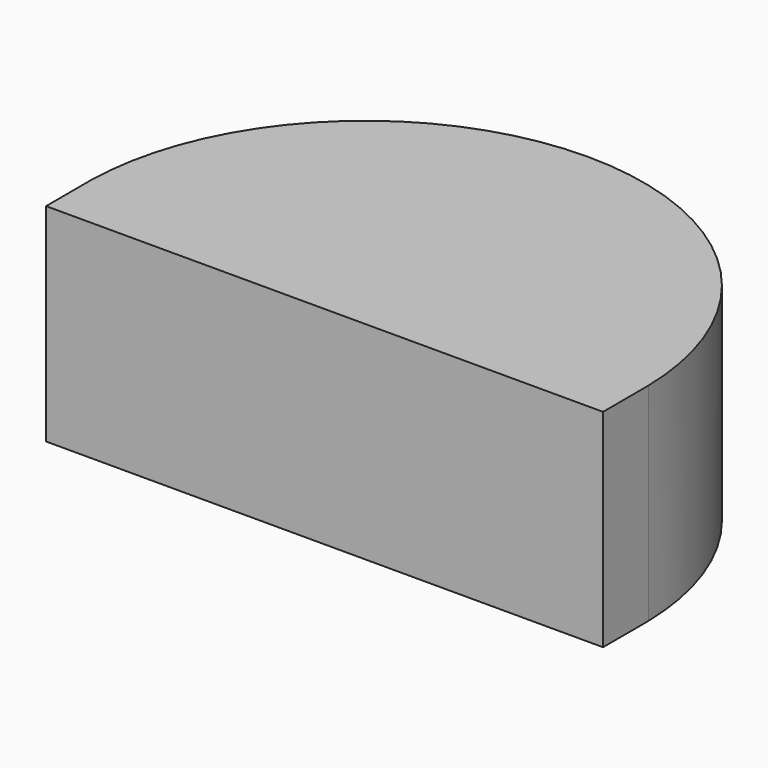
from build123d import *

# Parameters (mm, degrees)
F1_DEPTH = 25.4
F2_W     = 233.7879315019
F2_H     = 188.8666450977
F3_DEPTH = 91.948


# Not quite as in the source:
# - a feature names something its author has since deleted; it is built from what else it names


with BuildPart() as f1:
    # F0 (on Top) → F1 (new body)
    with BuildSketch(Plane.XY):
        with BuildLine():
            ThreePointArc((34.1941267741, -40.3357285894), (0.0107640733, -6.90975175), (-34.0682903974, -40.4420683952))
            Line((-34.0682903974, -40.4420683952), (-33.8233722324, -197.6617082131))
            Line((-33.8233722324, -197.6617082131), (34.4390449391, -197.5553684074))
            Line((34.4390449391, -197.5553684074), (34.1941267741, -40.3357285894))
        make_face()
    extrude(amount=F1_DEPTH)

    # F2 (on face) → F3 (cut)
    with BuildSketch(Plane(origin=(0, 0, 0), x_dir=(1, 0, 0), z_dir=(0, 0, -1))):
        with Locations((-8.5754804313, 141.7237520218)):
            Rectangle(F2_W, F2_H)
    extrude(amount=-F3_DEPTH, mode=Mode.SUBTRACT)


solid = f1.part
